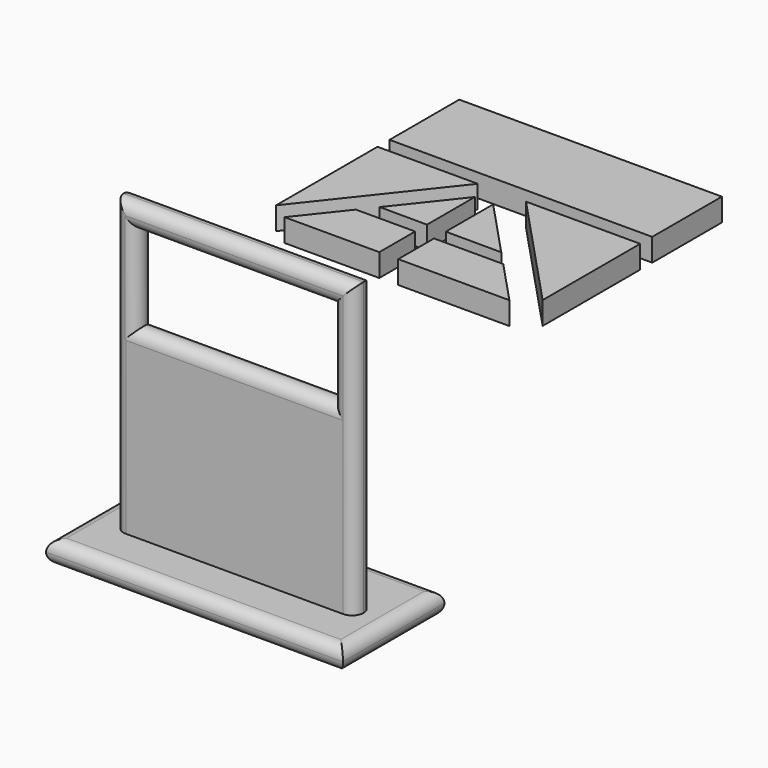
from build123d import *

# Parameters (mm, degrees)
F0_W          = 26.7775058746
F0_H          = 31.9101065397
F0_W_2        = 21.9197236001
F0_H_2        = 9.6741355956
F1_DEPTH      = 2.54
F2_DEPTH      = 2.54
F3_W          = 33.1266149879
F3_H          = 14.1676757485
F4_DEPTH      = 2.54
F6_W          = 29.3138232082
F6_H          = 9.7226984799
F7_DEPTH      = 2.54
F8_T1_DEPTH   = 33.1275058746
F8_T3_DEPTH   = 40.8001065397
F8_T5_DEPTH   = 9.6741355956
F8_T7_DEPTH   = 21.9197236001
F8_T13_DEPTH  = 12.8491355956
F8_T17_DEPTH  = 25.0947236001
F8_T24_DEPTH  = 12.8491355956
F8_T28_DEPTH  = 25.0947236001
F8_T35_DEPTH  = 25.0947236001
F8_T39_DEPTH  = 12.8491355956
F8_T46_DEPTH  = 12.8491355956
F8_T50_DEPTH  = 25.0947236001
F8_T57_DEPTH  = 25.0947236001
F8_T61_DEPTH  = 12.8491355956
F8_T68_DEPTH  = 25.0947236001
F8_T72_DEPTH  = 12.8491355956
F8_T79_DEPTH  = 12.8491355956
F8_T83_DEPTH  = 25.0947236001
F8_T90_DEPTH  = 25.0947236001
F8_T94_DEPTH  = 12.8491355956
F8_2_T1_DEPTH = 39.4766149879
F8_2_T3_DEPTH = 20.5176757485


# Not quite as in the source:
# - a fillet or chamfer that OpenCascade refuses, or shapes differently, is made with other operations: its cross-section is extruded or revolved along the edge and cut away or added


with BuildPart() as f1:
    # F0 (on Front) → F1 (new body)
    with BuildSketch(Plane.XZ):
        with Locations((0.6596446037, -1.20549649)):
            Rectangle(F0_W, F0_H)
        with Locations((0.5812961608, 7.34799169)):
            Rectangle(F0_W_2, F0_H_2, mode=Mode.SUBTRACT)
    extrude(amount=F1_DEPTH)

    # F2 (add): a face of the model
    f2_faces = [f1.faces().sort_by_distance(p)[0] for p in [
        (0.6596446037, -1.27, -17.1605497599),
    ]]
    extrude(f2_faces, amount=F2_DEPTH)

    # F8: fillet of radius 1.27 on 16 edges, made by hand

    # F8_s2 → F8_t1 (cut)
    with BuildSketch(Plane.YZ.offset(-15.9041083336)):
        with BuildLine():
            ThreePointArc((-1.27, 14.7495567799), (-2.1680256121, 14.377582392), (-2.54, 13.4795567799))
            Line((-2.54, 13.4795567799), (-2.54, 14.7495567799))
            Line((-2.54, 14.7495567799), (-1.27, 14.7495567799))
        make_face()
        with BuildLine():
            ThreePointArc((-2.54, -18.4305497599), (-2.1680256121, -19.328575372), (-1.27, -19.7005497599))
            Line((-1.27, -19.7005497599), (-2.54, -19.7005497599))
            Line((-2.54, -19.7005497599), (-2.54, -18.4305497599))
        make_face()
        with BuildLine():
            ThreePointArc((-1.27, 14.7495567799), (-0.3719743879, 14.377582392), (0, 13.4795567799))
            Line((0, 13.4795567799), (0, 14.7495567799))
            Line((0, 14.7495567799), (-1.27, 14.7495567799))
        make_face()
        with BuildLine():
            ThreePointArc((-1.27, -19.7005497599), (-0.3719743879, -19.328575372), (0, -18.4305497599))
            Line((0, -18.4305497599), (0, -19.7005497599))
            Line((0, -19.7005497599), (-1.27, -19.7005497599))
        make_face()
    extrude(amount=F8_T1_DEPTH, mode=Mode.SUBTRACT)

    # F8_s4 → F8_t3 (cut)
    with BuildSketch(Plane.XY.offset(-22.8755497599)):
        with BuildLine():
            ThreePointArc((-11.4591083336, -2.54), (-12.3571339457, -2.1680256121), (-12.7291083336, -1.27))
            Line((-12.7291083336, -1.27), (-12.7291083336, -2.54))
            Line((-12.7291083336, -2.54), (-11.4591083336, -2.54))
        make_face()
        with BuildLine():
            ThreePointArc((12.778397541, -2.54), (13.6764231532, -2.1680256121), (14.048397541, -1.27))
            Line((14.048397541, -1.27), (14.048397541, -2.54))
            Line((14.048397541, -2.54), (12.778397541, -2.54))
        make_face()
        with BuildLine():
            ThreePointArc((-11.4591083336, 0), (-12.3571339457, -0.3719743879), (-12.7291083336, -1.27))
            Line((-12.7291083336, -1.27), (-12.7291083336, 0))
            Line((-12.7291083336, 0), (-11.4591083336, 0))
        make_face()
        with BuildLine():
            ThreePointArc((12.778397541, 0), (13.6764231532, -0.3719743879), (14.048397541, -1.27))
            Line((14.048397541, -1.27), (14.048397541, 0))
            Line((14.048397541, 0), (12.778397541, 0))
        make_face()
    extrude(amount=F8_T3_DEPTH, mode=Mode.SUBTRACT)

    # F8_s6 → F8_t5 (cut)
    with BuildSketch(Plane.XY.offset(2.5109238923)):
        with BuildLine():
            ThreePointArc((-11.6485656393, -2.54), (-10.7505400272, -2.1680256121), (-10.3785656393, -1.27))
            Line((-10.3785656393, -1.27), (-10.3785656393, -2.54))
            Line((-10.3785656393, -2.54), (-11.6485656393, -2.54))
        make_face()
        with BuildLine():
            ThreePointArc((12.8111579609, -2.54), (11.9131323488, -2.1680256121), (11.5411579609, -1.27))
            Line((11.5411579609, -1.27), (11.5411579609, -2.54))
            Line((11.5411579609, -2.54), (12.8111579609, -2.54))
        make_face()
        with BuildLine():
            ThreePointArc((-10.3785656393, -1.27), (-10.7505400272, -0.3719743879), (-11.6485656393, 0))
            Line((-11.6485656393, 0), (-10.3785656393, 0))
            Line((-10.3785656393, 0), (-10.3785656393, -1.27))
        make_face()
        with BuildLine():
            ThreePointArc((11.5411579609, -1.27), (11.9131323488, -0.3719743879), (12.8111579609, 0))
            Line((12.8111579609, 0), (11.5411579609, 0))
            Line((11.5411579609, 0), (11.5411579609, -1.27))
        make_face()
    extrude(amount=F8_T5_DEPTH, mode=Mode.SUBTRACT)

    # F8_s8 → F8_t7 (cut)
    with BuildSketch(Plane.YZ.offset(-10.3785656393)):
        with BuildLine():
            ThreePointArc((-2.54, 13.4550594878), (-2.1680256121, 12.5570338757), (-1.27, 12.1850594878))
            Line((-1.27, 12.1850594878), (-2.54, 12.1850594878))
            Line((-2.54, 12.1850594878), (-2.54, 13.4550594878))
        make_face()
        with BuildLine():
            ThreePointArc((-2.54, 1.2409238923), (-2.1680256121, 2.1389495044), (-1.27, 2.5109238923))
            Line((-1.27, 2.5109238923), (-2.54, 2.5109238923))
            Line((-2.54, 2.5109238923), (-2.54, 1.2409238923))
        make_face()
        with BuildLine():
            ThreePointArc((-1.27, 12.1850594878), (-0.3719743879, 12.5570338757), (0, 13.4550594878))
            Line((0, 13.4550594878), (0, 12.1850594878))
            Line((0, 12.1850594878), (-1.27, 12.1850594878))
        make_face()
        with BuildLine():
            ThreePointArc((-1.27, 2.5109238923), (-0.3719743879, 2.1389495044), (0, 1.2409238923))
            Line((0, 1.2409238923), (0, 2.5109238923))
            Line((0, 2.5109238923), (-1.27, 2.5109238923))
        make_face()
    extrude(amount=F8_T7_DEPTH, mode=Mode.SUBTRACT)


with BuildPart() as f4:
    # F3 (on Top) → F4 (new body)
    with BuildSketch(Plane.XY):
        with Locations((0.3230758011, -0.609732233)):
            Rectangle(F3_W, F3_H)
    extrude(amount=F4_DEPTH)


with BuildPart() as f4_1:
    # F5: moved
    add(f4.part.moved(Location((0, 0, -20.3048437834))))

    # F8#2: fillet of radius 1.27 on 8 edges, made by hand

    # F8_2_s2 → F8_2_t1 (cut)
    with BuildSketch(Plane.YZ.offset(-19.4152316928)):
        with BuildLine():
            ThreePointArc((6.4741056412, -19.0348437834), (6.1021312534, -18.1368181713), (5.2041056412, -17.7648437834))
            Line((5.2041056412, -17.7648437834), (6.4741056412, -17.7648437834))
            Line((6.4741056412, -17.7648437834), (6.4741056412, -19.0348437834))
        make_face()
        with BuildLine():
            ThreePointArc((-7.6935701072, -19.0348437834), (-7.3215957193, -18.1368181713), (-6.4235701072, -17.7648437834))
            Line((-6.4235701072, -17.7648437834), (-7.6935701072, -17.7648437834))
            Line((-7.6935701072, -17.7648437834), (-7.6935701072, -19.0348437834))
        make_face()
        with BuildLine():
            ThreePointArc((6.4741056412, -19.0348437834), (6.1021312534, -19.9328693955), (5.2041056412, -20.3048437834))
            Line((5.2041056412, -20.3048437834), (6.4741056412, -20.3048437834))
            Line((6.4741056412, -20.3048437834), (6.4741056412, -19.0348437834))
        make_face()
        with BuildLine():
            ThreePointArc((-7.6935701072, -19.0348437834), (-7.3215957193, -19.9328693955), (-6.4235701072, -20.3048437834))
            Line((-6.4235701072, -20.3048437834), (-7.6935701072, -20.3048437834))
            Line((-7.6935701072, -20.3048437834), (-7.6935701072, -19.0348437834))
        make_face()
    extrude(amount=F8_2_T1_DEPTH, mode=Mode.SUBTRACT)

    # F8_2_s4 → F8_2_t3 (cut)
    with BuildSketch(Plane.XZ.offset(-9.6491056412)):
        with BuildLine():
            ThreePointArc((-16.2402316928, -19.0348437834), (-15.8682573049, -18.1368181713), (-14.9702316928, -17.7648437834))
            Line((-14.9702316928, -17.7648437834), (-16.2402316928, -17.7648437834))
            Line((-16.2402316928, -17.7648437834), (-16.2402316928, -19.0348437834))
        make_face()
        with BuildLine():
            ThreePointArc((16.8863832951, -19.0348437834), (16.5144089072, -18.1368181713), (15.6163832951, -17.7648437834))
            Line((15.6163832951, -17.7648437834), (16.8863832951, -17.7648437834))
            Line((16.8863832951, -17.7648437834), (16.8863832951, -19.0348437834))
        make_face()
        with BuildLine():
            ThreePointArc((-16.2402316928, -19.0348437834), (-15.8682573049, -19.9328693955), (-14.9702316928, -20.3048437834))
            Line((-14.9702316928, -20.3048437834), (-16.2402316928, -20.3048437834))
            Line((-16.2402316928, -20.3048437834), (-16.2402316928, -19.0348437834))
        make_face()
        with BuildLine():
            ThreePointArc((16.8863832951, -19.0348437834), (16.5144089072, -19.9328693955), (15.6163832951, -20.3048437834))
            Line((15.6163832951, -20.3048437834), (16.8863832951, -20.3048437834))
            Line((16.8863832951, -20.3048437834), (16.8863832951, -19.0348437834))
        make_face()
    extrude(amount=F8_2_T3_DEPTH, mode=Mode.SUBTRACT)


with BuildPart() as f7:
    # F6 (on Top) → F7 (new body)
    with BuildSketch(Plane.XY):
        with Locations((-0.937984325, 44.2727897316)):
            Rectangle(F6_W, F6_H)
    extrude(amount=F7_DEPTH)


with BuildPart() as f7b:
    # F6 (on Top) → F7, piece 2 (new body)
    with BuildSketch(Plane.XY):
        Polygon((-4.4132112525, 37.7321839333), (-15.5948959291, 37.7321839333), (-15.5948959291, 23.5834531486), align=None)
    extrude(amount=F7_DEPTH)


with BuildPart() as f7c:
    # F6 (on Top) → F7, piece 3 (new body)
    with BuildSketch(Plane.XY):
        Polygon((-3.0478241388, 28.9495810729), (-3.0478241388, 35.6352925301), (-8.334170212, 28.9674811065), align=None)
    extrude(amount=F7_DEPTH)


with BuildPart() as f7d:
    # F6 (on Top) → F7, piece 4 (new body)
    with BuildSketch(Plane.XY):
        Polygon((-9.6575162616, 27.2983089062), (-13.6205162853, 22.299669683), (-3.0478241388, 22.299669683), (-3.0478241388, 27.2983089062), align=None)
    extrude(amount=F7_DEPTH)


with BuildPart() as f7e:
    # F6 (on Top) → F7, piece 5 (new body)
    with BuildSketch(Plane.XY):
        Polygon((-0.937984325, 22.299669683), (11.4659758466, 22.299669683), (6.784225237, 27.2983089062), (-0.937984325, 27.2983089062), align=None)
    extrude(amount=F7_DEPTH)


with BuildPart() as f7f:
    # F6 (on Top) → F7, piece 6 (new body)
    with BuildSketch(Plane.XY):
        Polygon((5.2639957608, 28.9214365184), (-0.937984325, 35.5432033539), (-0.937984325, 28.9424369694), align=None)
    extrude(amount=F7_DEPTH)


with BuildPart() as f7g:
    # F6 (on Top) → F7, piece 7 (new body)
    with BuildSketch(Plane.XY):
        Polygon((13.7189272791, 24.1253394634), (13.7189272791, 37.7321839333), (0.9746883879, 37.7321839333), align=None)
    extrude(amount=F7_DEPTH)


with BuildPart() as f8_tool11:
    # F8_s12 → F8_t13 (new body)
    with BuildSketch(Plane.XY.offset(-0.6640761077)):
        with BuildLine():
            ThreePointArc((-11.6485656393, -2.54), (-10.7505400272, -2.1680256121), (-10.3785656393, -1.27))
            Line((-10.3785656393, -1.27), (-10.3785656393, -2.54))
            Line((-10.3785656393, -2.54), (-11.6485656393, -2.54))
        make_face()
    extrude(amount=F8_T13_DEPTH)

    split(bisect_by=Plane.XY.offset(2.5109238923), keep=Keep.BOTTOM)


with BuildPart() as f8_tool15:
    # F8_s16 → F8_t17 (new body)
    with BuildSketch(Plane.YZ.offset(11.5411579609)):
        with BuildLine():
            ThreePointArc((-2.54, 1.2409238923), (-2.1680256121, 2.1389495044), (-1.27, 2.5109238923))
            Line((-1.27, 2.5109238923), (-2.54, 2.5109238923))
            Line((-2.54, 2.5109238923), (-2.54, 1.2409238923))
        make_face()
    extrude(amount=-F8_T17_DEPTH)

    split(bisect_by=Plane.YZ.offset(-10.3785656393), keep=Keep.BOTTOM)


with BuildPart() as f8_tool11_1:
    add(f8_tool11.part)

    # F8_t19: intersect F8_tool15
    add(f8_tool15.part, mode=Mode.INTERSECT)


with BuildPart() as f1_1:
    add(f1.part)

    # F8_t9: cut F8_tool11
    add(f8_tool11_1.part, mode=Mode.SUBTRACT)


with BuildPart() as f8_tool22:
    # F8_s23 → F8_t24 (new body)
    with BuildSketch(Plane.XY.offset(2.5109238923)):
        with BuildLine():
            ThreePointArc((-11.6485656393, -2.54), (-10.7505400272, -2.1680256121), (-10.3785656393, -1.27))
            Line((-10.3785656393, -1.27), (-10.3785656393, -2.54))
            Line((-10.3785656393, -2.54), (-11.6485656393, -2.54))
        make_face()
    extrude(amount=F8_T24_DEPTH)

    split(bisect_by=Plane.XY.offset(12.1850594878), keep=Keep.TOP)


with BuildPart() as f8_tool26:
    # F8_s27 → F8_t28 (new body)
    with BuildSketch(Plane.YZ.offset(-13.5535656393)):
        with BuildLine():
            ThreePointArc((-2.54, 13.4550594878), (-2.1680256121, 12.5570338757), (-1.27, 12.1850594878))
            Line((-1.27, 12.1850594878), (-2.54, 12.1850594878))
            Line((-2.54, 12.1850594878), (-2.54, 13.4550594878))
        make_face()
    extrude(amount=F8_T28_DEPTH)

    split(bisect_by=Plane.YZ.offset(-10.3785656393), keep=Keep.BOTTOM)


with BuildPart() as f8_tool22_1:
    add(f8_tool22.part)

    # F8_t30: intersect F8_tool26
    add(f8_tool26.part, mode=Mode.INTERSECT)


with BuildPart() as f1_2:
    add(f1_1.part)

    # F8_t20: cut F8_tool22
    add(f8_tool22_1.part, mode=Mode.SUBTRACT)


with BuildPart() as f8_tool33:
    # F8_s34 → F8_t35 (new body)
    with BuildSketch(Plane.YZ.offset(-10.3785656393)):
        with BuildLine():
            ThreePointArc((-2.54, 13.4550594878), (-2.1680256121, 12.5570338757), (-1.27, 12.1850594878))
            Line((-1.27, 12.1850594878), (-2.54, 12.1850594878))
            Line((-2.54, 12.1850594878), (-2.54, 13.4550594878))
        make_face()
    extrude(amount=F8_T35_DEPTH)

    split(bisect_by=Plane.YZ.offset(11.5411579609), keep=Keep.TOP)


with BuildPart() as f8_tool37:
    # F8_s38 → F8_t39 (new body)
    with BuildSketch(Plane.XY.offset(15.3600594878)):
        with BuildLine():
            ThreePointArc((12.8111579609, -2.54), (11.9131323488, -2.1680256121), (11.5411579609, -1.27))
            Line((11.5411579609, -1.27), (11.5411579609, -2.54))
            Line((11.5411579609, -2.54), (12.8111579609, -2.54))
        make_face()
    extrude(amount=-F8_T39_DEPTH)

    split(bisect_by=Plane.XY.offset(12.1850594878), keep=Keep.TOP)


with BuildPart() as f8_tool33_1:
    add(f8_tool33.part)

    # F8_t41: intersect F8_tool37
    add(f8_tool37.part, mode=Mode.INTERSECT)


with BuildPart() as f1_3:
    add(f1_2.part)

    # F8_t31: cut F8_tool33
    add(f8_tool33_1.part, mode=Mode.SUBTRACT)


with BuildPart() as f8_tool44:
    # F8_s45 → F8_t46 (new body)
    with BuildSketch(Plane.XY.offset(12.1850594878)):
        with BuildLine():
            ThreePointArc((12.8111579609, -2.54), (11.9131323488, -2.1680256121), (11.5411579609, -1.27))
            Line((11.5411579609, -1.27), (11.5411579609, -2.54))
            Line((11.5411579609, -2.54), (12.8111579609, -2.54))
        make_face()
    extrude(amount=-F8_T46_DEPTH)

    split(bisect_by=Plane.XY.offset(2.5109238923), keep=Keep.BOTTOM)


with BuildPart() as f8_tool48:
    # F8_s49 → F8_t50 (new body)
    with BuildSketch(Plane.YZ.offset(14.7161579609)):
        with BuildLine():
            ThreePointArc((-2.54, 1.2409238923), (-2.1680256121, 2.1389495044), (-1.27, 2.5109238923))
            Line((-1.27, 2.5109238923), (-2.54, 2.5109238923))
            Line((-2.54, 2.5109238923), (-2.54, 1.2409238923))
        make_face()
    extrude(amount=-F8_T50_DEPTH)

    split(bisect_by=Plane.YZ.offset(11.5411579609), keep=Keep.TOP)


with BuildPart() as f8_tool44_1:
    add(f8_tool44.part)

    # F8_t52: intersect F8_tool48
    add(f8_tool48.part, mode=Mode.INTERSECT)


with BuildPart() as f1_4:
    add(f1_3.part)

    # F8_t42: cut F8_tool44
    add(f8_tool44_1.part, mode=Mode.SUBTRACT)


with BuildPart() as f8_tool55:
    # F8_s56 → F8_t57 (new body)
    with BuildSketch(Plane.YZ.offset(11.5411579609)):
        with BuildLine():
            ThreePointArc((-1.27, 2.5109238923), (-0.3719743879, 2.1389495044), (0, 1.2409238923))
            Line((0, 1.2409238923), (0, 2.5109238923))
            Line((0, 2.5109238923), (-1.27, 2.5109238923))
        make_face()
    extrude(amount=-F8_T57_DEPTH)

    split(bisect_by=Plane.YZ.offset(-10.3785656393), keep=Keep.BOTTOM)


with BuildPart() as f8_tool59:
    # F8_s60 → F8_t61 (new body)
    with BuildSketch(Plane.XY.offset(-0.6640761077)):
        with BuildLine():
            ThreePointArc((-10.3785656393, -1.27), (-10.7505400272, -0.3719743879), (-11.6485656393, 0))
            Line((-11.6485656393, 0), (-10.3785656393, 0))
            Line((-10.3785656393, 0), (-10.3785656393, -1.27))
        make_face()
    extrude(amount=F8_T61_DEPTH)

    split(bisect_by=Plane.XY.offset(2.5109238923), keep=Keep.BOTTOM)


with BuildPart() as f8_tool55_1:
    add(f8_tool55.part)

    # F8_t63: intersect F8_tool59
    add(f8_tool59.part, mode=Mode.INTERSECT)


with BuildPart() as f1_5:
    add(f1_4.part)

    # F8_t53: cut F8_tool55
    add(f8_tool55_1.part, mode=Mode.SUBTRACT)


with BuildPart() as f8_tool66:
    # F8_s67 → F8_t68 (new body)
    with BuildSketch(Plane.YZ.offset(-13.5535656393)):
        with BuildLine():
            ThreePointArc((-1.27, 12.1850594878), (-0.3719743879, 12.5570338757), (0, 13.4550594878))
            Line((0, 13.4550594878), (0, 12.1850594878))
            Line((0, 12.1850594878), (-1.27, 12.1850594878))
        make_face()
    extrude(amount=F8_T68_DEPTH)

    split(bisect_by=Plane.YZ.offset(-10.3785656393), keep=Keep.BOTTOM)


with BuildPart() as f8_tool70:
    # F8_s71 → F8_t72 (new body)
    with BuildSketch(Plane.XY.offset(2.5109238923)):
        with BuildLine():
            ThreePointArc((-10.3785656393, -1.27), (-10.7505400272, -0.3719743879), (-11.6485656393, 0))
            Line((-11.6485656393, 0), (-10.3785656393, 0))
            Line((-10.3785656393, 0), (-10.3785656393, -1.27))
        make_face()
    extrude(amount=F8_T72_DEPTH)

    split(bisect_by=Plane.XY.offset(12.1850594878), keep=Keep.TOP)


with BuildPart() as f8_tool66_1:
    add(f8_tool66.part)

    # F8_t74: intersect F8_tool70
    add(f8_tool70.part, mode=Mode.INTERSECT)


with BuildPart() as f1_6:
    add(f1_5.part)

    # F8_t64: cut F8_tool66
    add(f8_tool66_1.part, mode=Mode.SUBTRACT)


with BuildPart() as f8_tool77:
    # F8_s78 → F8_t79 (new body)
    with BuildSketch(Plane.XY.offset(15.3600594878)):
        with BuildLine():
            ThreePointArc((11.5411579609, -1.27), (11.9131323488, -0.3719743879), (12.8111579609, 0))
            Line((12.8111579609, 0), (11.5411579609, 0))
            Line((11.5411579609, 0), (11.5411579609, -1.27))
        make_face()
    extrude(amount=-F8_T79_DEPTH)

    split(bisect_by=Plane.XY.offset(12.1850594878), keep=Keep.TOP)


with BuildPart() as f8_tool81:
    # F8_s82 → F8_t83 (new body)
    with BuildSketch(Plane.YZ.offset(-10.3785656393)):
        with BuildLine():
            ThreePointArc((-1.27, 12.1850594878), (-0.3719743879, 12.5570338757), (0, 13.4550594878))
            Line((0, 13.4550594878), (0, 12.1850594878))
            Line((0, 12.1850594878), (-1.27, 12.1850594878))
        make_face()
    extrude(amount=F8_T83_DEPTH)

    split(bisect_by=Plane.YZ.offset(11.5411579609), keep=Keep.TOP)


with BuildPart() as f8_tool77_1:
    add(f8_tool77.part)

    # F8_t85: intersect F8_tool81
    add(f8_tool81.part, mode=Mode.INTERSECT)


with BuildPart() as f1_7:
    add(f1_6.part)

    # F8_t75: cut F8_tool77
    add(f8_tool77_1.part, mode=Mode.SUBTRACT)


with BuildPart() as f8_tool88:
    # F8_s89 → F8_t90 (new body)
    with BuildSketch(Plane.YZ.offset(14.7161579609)):
        with BuildLine():
            ThreePointArc((-1.27, 2.5109238923), (-0.3719743879, 2.1389495044), (0, 1.2409238923))
            Line((0, 1.2409238923), (0, 2.5109238923))
            Line((0, 2.5109238923), (-1.27, 2.5109238923))
        make_face()
    extrude(amount=-F8_T90_DEPTH)

    split(bisect_by=Plane.YZ.offset(11.5411579609), keep=Keep.TOP)


with BuildPart() as f8_tool92:
    # F8_s93 → F8_t94 (new body)
    with BuildSketch(Plane.XY.offset(12.1850594878)):
        with BuildLine():
            ThreePointArc((11.5411579609, -1.27), (11.9131323488, -0.3719743879), (12.8111579609, 0))
            Line((12.8111579609, 0), (11.5411579609, 0))
            Line((11.5411579609, 0), (11.5411579609, -1.27))
        make_face()
    extrude(amount=-F8_T94_DEPTH)

    split(bisect_by=Plane.XY.offset(2.5109238923), keep=Keep.BOTTOM)


with BuildPart() as f8_tool88_1:
    add(f8_tool88.part)

    # F8_t96: intersect F8_tool92
    add(f8_tool92.part, mode=Mode.INTERSECT)


with BuildPart() as f1_8:
    add(f1_7.part)

    # F8_t86: cut F8_tool88
    add(f8_tool88_1.part, mode=Mode.SUBTRACT)


solid = Compound([f4_1.part, f7.part, f7b.part, f7c.part, f7d.part, f7e.part, f7f.part, f7g.part, f1_8.part])
